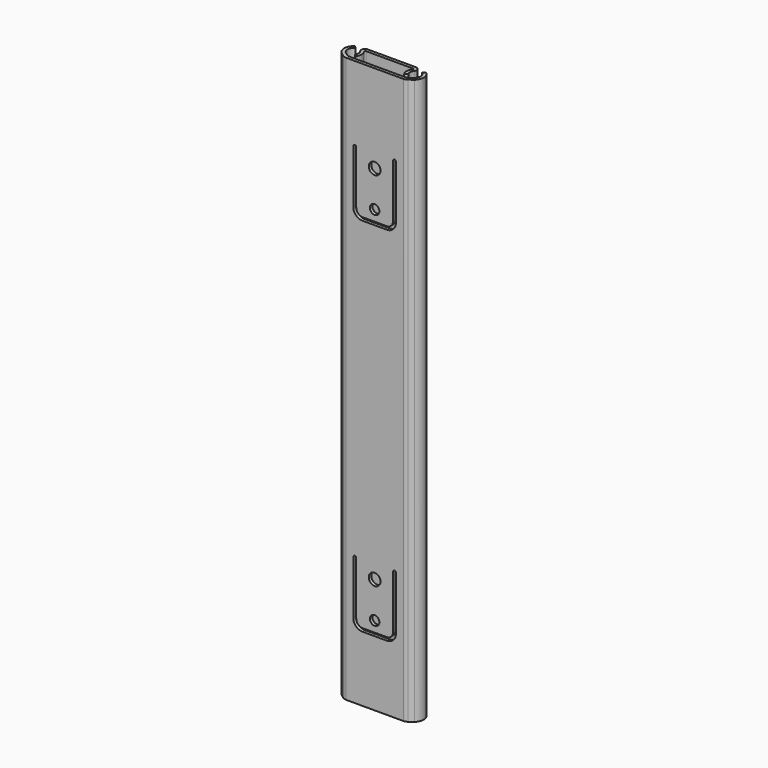
from build123d import *

# Parameters (mm, degrees)
F2_DEPTH     = 250
F3_DEPTH     = 250
F4_W         = 4.5
F4_H         = 9.2
F5_DEPTH     = 25
F4_W_2       = 9.2
F4_H_2       = 4.5
F4_R         = 2.25
F8_R         = 2.24999
F8_2_R       = 2.24999
F14_DEPTH    = 6
F13_R        = 2.1
F13_R_2      = 2.6
F15_R        = 4
F16_R        = 2.8
F17_T1_DEPTH = 9.5


# Not quite as in the source:
# - a fillet or chamfer that OpenCascade refuses, or shapes differently, is made with other operations: its cross-section is extruded or revolved along the edge and cut away or added
# - a fillet or chamfer is up to 0.001 mm smaller than in the source, because OpenCascade refuses the exact size


with BuildPart() as f2:
    # F1 (on Top) → F2 (new body)
    with BuildSketch(Plane.XY):
        with BuildLine():
            Line((-11.8238357827, -0.8677195292), (-10.7275778428, -1.8694410791))
            ThreePointArc((-10.7275778428, -1.8694410791), (-9.9382011717, 0.3618114698), (-10.5848610401, 2.6385271922))
            ThreePointArc((-10.5848610401, 2.6385271922), (-10.6721948967, 3.1240050413), (-10.2586513385, 3.3928873017))
            Line((-10.2586513385, 3.3928873017), (10.5257425457, 3.3928873017))
            ThreePointArc((10.5257425457, 3.3928873017), (10.8736199043, 3.1365507058), (10.731831193, 2.7283558156))
            ThreePointArc((10.731831193, 2.7283558156), (9.9471667751, 0.455322268), (10.731831193, -1.8177112797))
            Line((10.731831193, -1.8177112797), (11.8592558429, -0.8600065485))
            ThreePointArc((11.8592558429, -0.8600065485), (11.3668469211, 0.6546838766), (11.9562381878, 2.1343363915))
            ThreePointArc((11.9562381878, 2.1343363915), (12.1496041237, 2.7488216154), (12.1623268351, 3.3928873017))
            ThreePointArc((12.1623268351, 3.3928873017), (11.7162853066, 4.4052676185), (10.6833400205, 4.8013622873))
            Line((10.6833400205, 4.8013622873), (-10.7308318838, 4.8013622873))
            ThreePointArc((-10.7308318838, 4.8013622873), (-11.7888176914, 4.3568184571), (-12.2117670253, 3.2900162041))
            ThreePointArc((-12.2117670253, 3.2900162041), (-12.1485508104, 2.6137193167), (-11.8238357827, 2.0171173383))
            ThreePointArc((-11.8238357827, 2.0171173383), (-11.3595728447, 0.5746989045), (-11.8238357827, -0.8677195292))
        make_face()
    extrude(amount=F2_DEPTH)


with BuildPart() as f3:
    # F1 (on Top) → F3 (new body)
    with BuildSketch(Plane.XY):
        with BuildLine():
            ThreePointArc((-15.040784136, -1.8694410791), (-16.1252354526, 0.6606326234), (-14.6316215396, 2.9728664085))
            Line((-14.6316215396, 2.9728664085), (-15.6602784991, 3.9672353305))
            ThreePointArc((-15.6602784991, 3.9672353305), (-17.5947215903, 0.617735278), (-16.0031653941, -2.9076256324))
            Line((-16.0031653941, -2.9076256324), (-14.5143490806, -4.0940172111))
            ThreePointArc((-14.5143490806, -4.0940172111), (-13.5937394916, -4.5972187997), (-12.5571619719, -4.7592092305))
            Line((-12.5571619719, -4.7592092305), (12.7876326442, -4.7592092305))
            ThreePointArc((12.7876326442, -4.7592092305), (13.5980508192, -4.6201771633), (14.3157895654, -4.21898067))
            Line((14.3157895654, -4.21898067), (16.1611102521, -2.863822272))
            ThreePointArc((16.1611102521, -2.863822272), (17.5805681578, 0.6595379776), (15.7430302352, 3.9840503596))
            Line((15.7430302352, 3.9840503596), (14.7194536403, 2.9460568912))
            ThreePointArc((14.7194536403, 2.9460568912), (16.1669970409, 0.6050832532), (15.0222023949, -1.8979118904))
            Line((15.0222023949, -1.8979118904), (13.7213492466, -2.8877414463))
            ThreePointArc((13.7213492466, -2.8877414463), (13.1343028227, -3.2124911979), (12.4788619578, -3.35561065))
            Line((12.4788619578, -3.35561065), (-12.2050791979, -3.35561065))
            ThreePointArc((-12.2050791979, -3.35561065), (-12.8698089882, -3.2539225108), (-13.4737379849, -2.9581591953))
            Line((-13.4737379849, -2.9581591953), (-15.040784136, -1.8694410791))
        make_face()
    extrude(amount=F3_DEPTH)


with BuildPart() as f5:
    # F4 (on face) → F5 (new body)
    with BuildSketch(Plane.XZ.offset(4.7592092305)):
        with Locations((0, 37)):
            Rectangle(F4_W, F4_H)
    extrude(amount=F5_DEPTH)


with BuildPart() as f5b:
    # F4 (on face) → F5, piece 2 (new body)
    with BuildSketch(Plane.XZ.offset(4.7592092305)):
        with Locations((0, 53)):
            Rectangle(F4_W_2, F4_H_2)
    extrude(amount=F5_DEPTH)


with BuildPart() as f5c:
    # F4 (on face) → F5, piece 3 (new body)
    with BuildSketch(Plane.XZ.offset(4.7592092305)):
        with Locations((0, 62)):
            Circle(F4_R)
    extrude(amount=F5_DEPTH)


with BuildPart() as f5d:
    # F4 (on face) → F5, piece 4 (new body)
    with BuildSketch(Plane.XZ.offset(4.7592092305)):
        with Locations((0, 229)):
            Circle(F4_R)
    extrude(amount=F5_DEPTH)


with BuildPart() as f5d_1:
    # F6: moved
    add(f5d.part.moved(Location((0, 29, 0))))


with BuildPart() as f5c_1:
    # F6: moved
    add(f5c.part.moved(Location((0, 29, 0))))


with BuildPart() as f5b_1:
    # F6: moved
    add(f5b.part.moved(Location((0, 29, 0))))


with BuildPart() as f5_1:
    # F6: moved
    add(f5.part.moved(Location((0, 29, 0))))


with BuildPart() as f5d_2:
    # F7: moved
    add(f5d_1.part.moved(Location((0, 2.4, 0))))


with BuildPart() as f5c_2:
    # F7: moved
    add(f5c_1.part.moved(Location((0, 2.4, 0))))


with BuildPart() as f5b_2:
    # F7: moved
    add(f5b_1.part.moved(Location((0, 2.4, 0))))

    # F8 (radius 2.25 in the source; OpenCascade refuses exactly that, so slightly less here)
    f8_edges = [f5b_2.edges().sort_by_distance(p)[0] for p in [
        (-4.6, 14.140791, 50.75),
        (4.6, 14.140791, 50.75),
        (-4.6, 14.140791, 55.25),
        (4.6, 14.140791, 55.25),
    ]]
    fillet(f8_edges, radius=F8_R)


with BuildPart() as f5_2:
    # F7: moved
    add(f5_1.part.moved(Location((0, 2.4, 0))))

    # F8#2 (radius 2.25 in the source; OpenCascade refuses exactly that, so slightly less here)
    f8_2_edges = [f5_2.edges().sort_by_distance(p)[0] for p in [
        (-2.25, 14.140791, 41.6),
        (-2.25, 14.140791, 32.4),
        (2.25, 14.140791, 32.4),
        (2.25, 14.140791, 41.6),
    ]]
    fillet(f8_2_edges, radius=F8_2_R)


with BuildPart() as f2_1:
    add(f2.part)

    # F9: cut F5
    add(f5_2.part, mode=Mode.SUBTRACT)

    # F10: cut F5d
    add(f5d_2.part, mode=Mode.SUBTRACT)

    # F11: cut F5b
    add(f5b_2.part, mode=Mode.SUBTRACT)

    # F12: cut F5c
    add(f5c_2.part, mode=Mode.SUBTRACT)


with BuildPart() as f14:
    # F13 (on Front) → F14 (new body)
    with BuildSketch(Plane.XZ):
        Polygon((-9.4226980582, 28.8961585611), (0, 28.8961585611), (0, 30.2952826023), (-8.1285946071, 30.2952826023), (-8.1285946071, 57.3633499444), (-9.4226980582, 57.3633499444), align=None)
        Polygon((0, 30.2952826023), (0, 28.8961585611), (9.4226980582, 28.8961585611), (9.4226980582, 57.3633499444), (8.1285946071, 57.3633499444), (8.1285946071, 30.2952826023), align=None)
    extrude(amount=F14_DEPTH)

    # F15
    f15_edges = [f14.edges().sort_by_distance(p)[0] for p in [
        (9.422698, -3, 28.896159),
        (-9.422698, -3, 28.896159),
    ]]
    fillet(f15_edges, radius=F15_R)

    # F16
    f16_edges = [f14.edges().sort_by_distance(p)[0] for p in [
        (-8.128595, -3, 30.295283),
        (8.128595, -3, 30.295283),
    ]]
    fillet(f16_edges, radius=F16_R)

    # F17: fillet of radius 0.7 on 4 edges, made by hand

    # F17_s2 → F17_t1 (cut)
    with BuildSketch(Plane.XZ.offset(-1.75)):
        with BuildLine():
            ThreePointArc((-8.1285946071, 56.6633499444), (-8.3336198603, 57.1583246912), (-8.8285946071, 57.3633499444))
            Line((-8.8285946071, 57.3633499444), (-8.1285946071, 57.3633499444))
            Line((-8.1285946071, 57.3633499444), (-8.1285946071, 56.6633499444))
        make_face()
        with BuildLine():
            ThreePointArc((-8.7226980582, 57.3633499444), (-9.217672805, 57.1583246912), (-9.4226980582, 56.6633499444))
            Line((-9.4226980582, 56.6633499444), (-9.4226980582, 57.3633499444))
            Line((-9.4226980582, 57.3633499444), (-8.7226980582, 57.3633499444))
        make_face()
        with BuildLine():
            ThreePointArc((8.1285946071, 56.6633499444), (8.3336198603, 57.1583246912), (8.8285946071, 57.3633499444))
            Line((8.8285946071, 57.3633499444), (8.1285946071, 57.3633499444))
            Line((8.1285946071, 57.3633499444), (8.1285946071, 56.6633499444))
        make_face()
        with BuildLine():
            ThreePointArc((8.7226980582, 57.3633499444), (9.217672805, 57.1583246912), (9.4226980582, 56.6633499444))
            Line((9.4226980582, 56.6633499444), (9.4226980582, 57.3633499444))
            Line((9.4226980582, 57.3633499444), (8.7226980582, 57.3633499444))
        make_face()
    extrude(amount=F17_T1_DEPTH, mode=Mode.SUBTRACT)


with BuildPart() as f14b:
    # F13 (on Front) → F14, piece 2 (new body)
    with BuildSketch(Plane.XZ):
        with Locations((0, 35)):
            Circle(F13_R)
    extrude(amount=F14_DEPTH)


with BuildPart() as f14c:
    # F13 (on Front) → F14, piece 3 (new body)
    with BuildSketch(Plane.XZ):
        with Locations((0, 51)):
            Circle(F13_R_2)
    extrude(amount=F14_DEPTH)


with BuildPart() as f18_1:
    # F18: copy of F14b
    add(f14b.part.moved(Location((0, 0, 97))))


with BuildPart() as f18_2:
    # F18: copy of F14c
    add(f14c.part.moved(Location((0, 0, 97))))


with BuildPart() as f18_3:
    # F18: copy of F14
    add(f14.part.moved(Location((0, 0, 97))))


with BuildPart() as f18_2_1:
    # F19: moved
    add(f18_2.part.moved(Location((0, 0, 63))))


with BuildPart() as f18_1_1:
    # F19: moved
    add(f18_1.part.moved(Location((0, 0, 63))))


with BuildPart() as f18_3_1:
    # F19: moved
    add(f18_3.part.moved(Location((0, 0, 63))))


with BuildPart() as f3_1:
    add(f3.part)

    # F20: cut F18_1, F14, F14c, F18_2, F18_3, F14b
    add(f18_1_1.part, mode=Mode.SUBTRACT)
    add(f14.part, mode=Mode.SUBTRACT)
    add(f14c.part, mode=Mode.SUBTRACT)
    add(f18_2_1.part, mode=Mode.SUBTRACT)
    add(f18_3_1.part, mode=Mode.SUBTRACT)
    add(f14b.part, mode=Mode.SUBTRACT)


solid = Compound([f2_1.part, f3_1.part])
